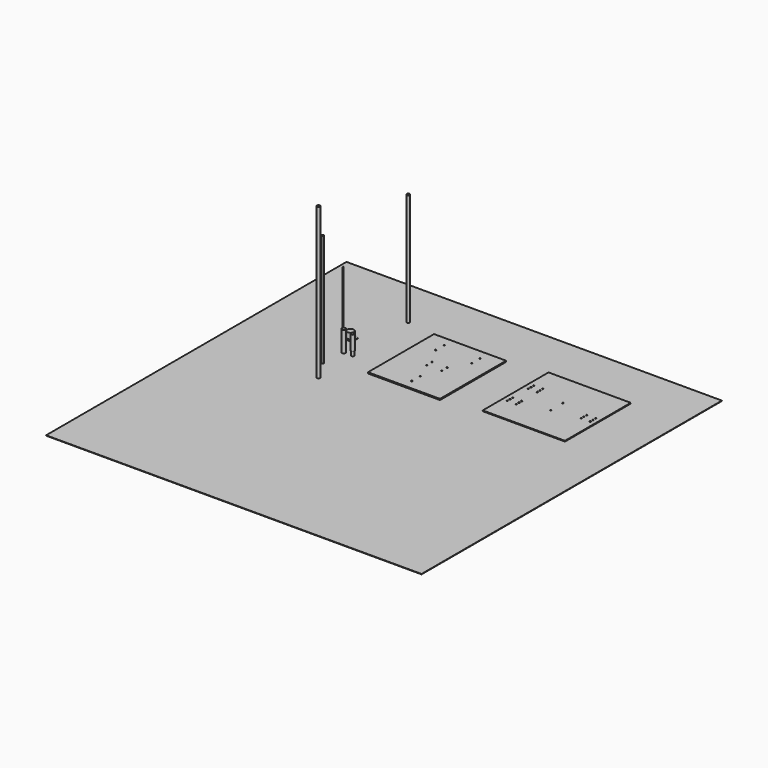
from build123d import *

# Parameters (mm, degrees)
F0_R      = 1.7
F1_DEPTH  = 4
F2_R      = 4
F3_DEPTH  = 300
F4_W      = 1000
F4_H      = 1000
F5_DEPTH  = 1
F6_R      = 4
F7_DEPTH  = 403
F6_R_2    = 2.5
F8_DEPTH  = 300
F6_R_3    = 9
F9_DEPTH  = 17.5
F10_DEPTH = 2
F6_R_4    = 5
F11_DEPTH = 56
F12_START = 13
F12_DEPTH = 39
F13_DEPTH = 52
F14_W     = 219
F14_H     = 219
F14_R     = 1.7
F15_DEPTH = 3
F2_R_2    = 0.875
F16_DEPTH = 150
F14_R_2   = 1.5
F17_DEPTH = 3


with BuildPart() as f1:
    # F0 (on Top) → F1 (new body)
    with BuildSketch(Plane.XY):
        Polygon((-139.0947423129, 71.8948530406), (-139.0947423129, -148.1051469594), (52.7424413346, -148.1051469594), (52.7424413346, 71.8948530406), (-44.1732802409, 71.8264897118), align=None)
        with Locations((-63.7154691358, -47.1051469594)):
            Circle(F0_R, mode=Mode.SUBTRACT)
        with Locations((-43.1761504892, -122.1051469594)):
            Circle(F0_R, mode=Mode.SUBTRACT)
        with Locations((-43.1761504892, -94.1051469594)):
            Circle(F0_R, mode=Mode.SUBTRACT)
        with Locations((-23.7154691358, -47.1051469594)):
            Circle(F0_R, mode=Mode.SUBTRACT)
        with Locations((-63.7154691358, -29.1051469594)):
            Circle(F0_R, mode=Mode.SUBTRACT)
        with Locations((-91.6340112769, 17.8606713762)):
            Circle(F0_R, mode=Mode.SUBTRACT)
        with Locations((-91.6340112769, 45.8606713762)):
            Circle(F0_R, mode=Mode.SUBTRACT)
        with Locations((-23.7154691358, -29.1051469594)):
            Circle(F0_R, mode=Mode.SUBTRACT)
        with Locations((4.2845805468, 17.8606713762)):
            Circle(F0_R, mode=Mode.SUBTRACT)
        with Locations((4.2845805468, 45.8606713762)):
            Circle(F0_R, mode=Mode.SUBTRACT)
    extrude(amount=F1_DEPTH)


with BuildPart() as f3:
    # F2 (on Top) → F3 (new body)
    with BuildSketch(Plane.XY):
        with Locations((-218.4958606958, 85.2202251554)):
            Circle(F2_R)
    extrude(amount=F3_DEPTH)


with BuildPart() as f5:
    # F4 (on Top) → F5 (new body)
    with BuildSketch(Plane.XY):
        with Locations((11.9614601135, -283.5388973286)):
            Rectangle(F4_W, F4_H)
    extrude(amount=F5_DEPTH)


with BuildPart() as f7:
    # F6 (on Top) → F7 (new body)
    with BuildSketch(Plane.XY):
        with Locations((-208.2721143961, -226.4990210533)):
            Circle(F6_R)
    extrude(amount=F7_DEPTH)


with BuildPart() as f8:
    # F6 (on Top) → F8 (new body)
    with BuildSketch(Plane.XY):
        with Locations((-241.9700175524, -169.9271649122)):
            Circle(F6_R_2)
    extrude(amount=F8_DEPTH)


with BuildPart() as f9:
    # F6 (on Top) → F9 (new body, symmetric)
    with BuildSketch(Plane.XY):
        with Locations((-267.6430344582, -45.3749746084)):
            Circle(F6_R_3)
    extrude(amount=F9_DEPTH, both=True)

    # F6 (on Top) → F10 (join)
    with BuildSketch(Plane.XY):
        Polygon((-281.1430344582, -37.5807459744), (-281.1430344582, -53.1692032425), (-267.6430344582, -60.9634318765), (-254.1430344582, -53.1692032425), (-254.1430344582, -37.5807459744), (-267.6430344582, -29.7865173403), align=None)
        with Locations((-267.6430344582, -45.3749746084)):
            Circle(F6_R_3, mode=Mode.SUBTRACT)
    extrude(amount=F10_DEPTH)


with BuildPart() as f11:
    # F6 (on Top) → F11 (new body)
    with BuildSketch(Plane.XY):
        with Locations((-238.0250245333, -104.8983484507)):
            Circle(F6_R_4)
    extrude(amount=F11_DEPTH)


with BuildPart() as f12:
    # F6 (on Top) → F12 (new body)
    with BuildSketch(Plane.XY.offset(F12_START)):
        with Locations((-214.7895480695, -104.3171395545)):
            Circle(F6_R_4)
        with Locations((-214.7895480695, -104.3171395545)):
            Circle(F6_R, mode=Mode.SUBTRACT)
    extrude(amount=F12_DEPTH)

    # F6 (on Top) → F13 (join)
    with BuildSketch(Plane.XY):
        with Locations((-214.7895480695, -104.3171395545)):
            Circle(F6_R)
    extrude(amount=F13_DEPTH)


with BuildPart() as f15:
    # F14 (on Top) → F15 (new body)
    with BuildSketch(Plane.XY):
        with Locations((262.9949003458, -22.268660448)):
            Rectangle(F14_W, F14_H)
        with Locations((166.4949003458, -66.268660448)):
            Circle(F14_R, mode=Mode.SUBTRACT)
        with Locations((190.4949003458, -66.268660448)):
            Circle(F14_R, mode=Mode.SUBTRACT)
        with Locations((166.4949003458, -57.268660448)):
            Circle(F14_R, mode=Mode.SUBTRACT)
        with Locations((190.4949003458, -57.268660448)):
            Circle(F14_R, mode=Mode.SUBTRACT)
        with Locations((166.4949003458, -48.268660448)):
            Circle(F14_R, mode=Mode.SUBTRACT)
        with Locations((190.4949003458, -48.268660448)):
            Circle(F14_R, mode=Mode.SUBTRACT)
        with Locations((262.9949003458, -42.768660448)):
            Circle(F14_R, mode=Mode.SUBTRACT)
        with Locations((335.4949003458, -31.268660448)):
            Circle(F14_R, mode=Mode.SUBTRACT)
        with Locations((359.4949003458, -31.268660448)):
            Circle(F14_R, mode=Mode.SUBTRACT)
        with Locations((166.4949003458, 3.731339552)):
            Circle(F14_R, mode=Mode.SUBTRACT)
        with Locations((190.4949003458, 3.731339552)):
            Circle(F14_R, mode=Mode.SUBTRACT)
        with Locations((166.4949003458, 12.731339552)):
            Circle(F14_R, mode=Mode.SUBTRACT)
        with Locations((190.4949003458, 12.731339552)):
            Circle(F14_R, mode=Mode.SUBTRACT)
        with Locations((166.4949003458, 21.731339552)):
            Circle(F14_R, mode=Mode.SUBTRACT)
        with Locations((190.4949003458, 21.731339552)):
            Circle(F14_R, mode=Mode.SUBTRACT)
        with Locations((262.9949003458, -1.768660448)):
            Circle(F14_R, mode=Mode.SUBTRACT)
        with Locations((335.4949003458, -22.268660448)):
            Circle(F14_R, mode=Mode.SUBTRACT)
        with Locations((359.4949003458, -22.268660448)):
            Circle(F14_R, mode=Mode.SUBTRACT)
        with Locations((335.4949003458, -13.268660448)):
            Circle(F14_R, mode=Mode.SUBTRACT)
        with Locations((359.4949003458, -13.268660448)):
            Circle(F14_R, mode=Mode.SUBTRACT)
    extrude(amount=F15_DEPTH)


with BuildPart() as f16:
    # F2 (on Top) → F16 (new body)
    with BuildSketch(Plane.XY):
        with Locations((-300.4790842533, -29.0999822319)):
            Circle(F2_R_2)
    extrude(amount=F16_DEPTH)


with BuildPart() as f17:
    # F14 (on Top) → F17 (new body)
    with BuildSketch(Plane.XY):
        with Locations((-295.1983672105, -29.0999822319)):
            Circle(F14_R_2)
    extrude(amount=-F17_DEPTH)


solid = Compound([f1.part, f3.part, f5.part, f7.part, f8.part, f9.part, f11.part, f12.part, f15.part, f16.part, f17.part])
